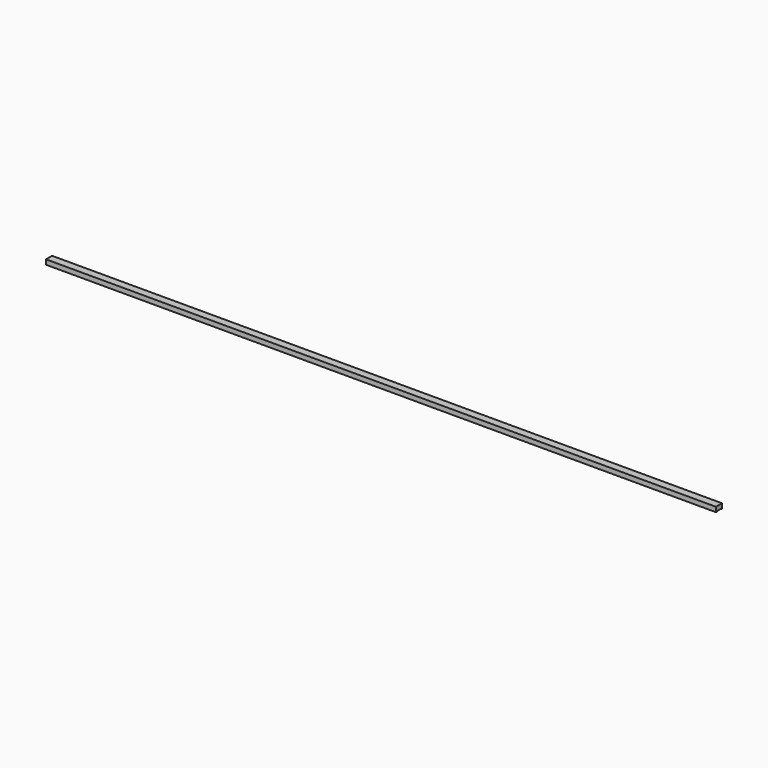
from build123d import *

# Parameters (mm, degrees)
F1_DEPTH = 10840


with BuildPart() as f1:
    # F0 (on Right) → F1 (new body)
    with BuildSketch(Plane.YZ):
        Polygon((-18, 0), (0, 0), (0, 80), (-120, 77.6), (-120, 0), (-102, 0), (-102, 8), (-18, 8), align=None)
    extrude(amount=F1_DEPTH)


solid = f1.part
